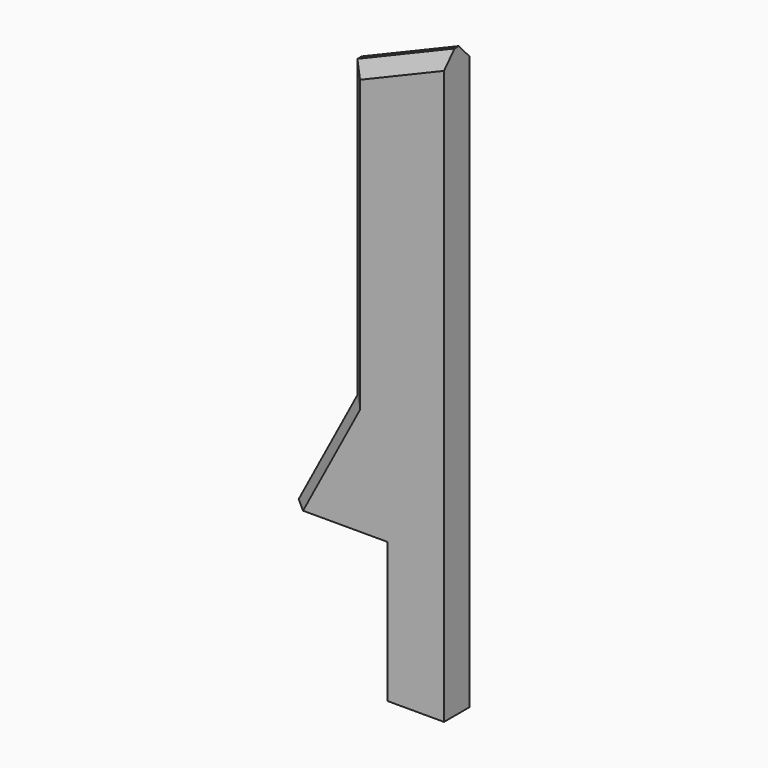
from build123d import *

# Parameters (mm, degrees)
F1_DEPTH = 6.096
F3_SIZE  = 2.54


# Not quite as in the source:
# - a feature of the source that left no trace in its solid (it failed there, or was rolled back) is left out


with BuildPart() as f1:
    # F0 (on Front) → F1 (new body)
    with BuildSketch(Plane.XZ):
        Polygon((0, 0), (0, 64.7907108068), (-18.6979882419, 56.9636411965), (-18.6979882419, 0), align=None)
        Polygon((0, -48.266902566), (0, 0), (-18.6979882419, 0), (-30.0037488341, -21.3070102036), (-10.8709232882, -21.3070102036), (-10.8709232882, -48.266902566), align=None)
    extrude(amount=F1_DEPTH)

    # F3
    f3_edges = [f1.edges().sort_by_distance(p)[0] for p in [
        (-18.697988, -6.096, 28.481821),
        (-24.350869, -6.096, -10.653505),
        (-9.348994, -6.096, 60.877176),
        (-9.348994, 0, 60.877176),
        (-18.697988, 0, 28.481821),
        (-24.350869, 0, -10.653505),
    ]]
    chamfer(f3_edges, length=F3_SIZE)


solid = f1.part
